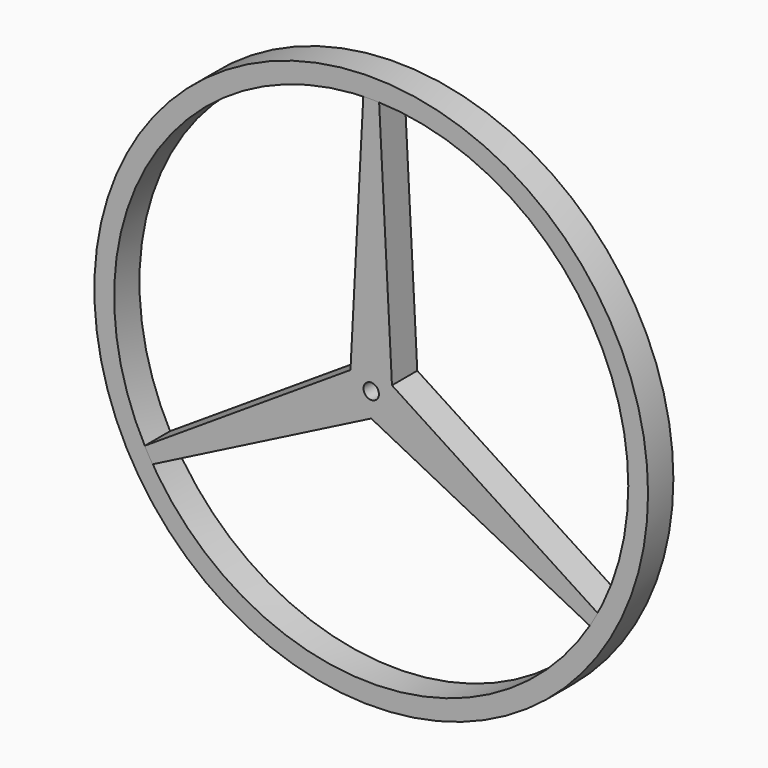
from build123d import *

# Parameters (mm, degrees)
F0_R     = 35
F0_R_2   = 32.5
F1_DEPTH = 4
F0_R_3   = 2.975
F0_R_4   = 0.975
F3_DEPTH = 4


with BuildPart() as f1:
    # F0 (on Front) → F1 (new body)
    with BuildSketch(Plane.XZ):
        Circle(F0_R)
        Circle(F0_R_2, mode=Mode.SUBTRACT)
    extrude(amount=F1_DEPTH)

    # F4 (on Right) → F5 (revolve, cut)
    with BuildSketch(Plane.YZ):
        Polygon((0, 32.5291901827), (2.1413064096, 1.5684039099), (5.6291026995, 1.5684039099), (5.6291026995, 33.8882990181), (0, 33.8882990181), align=None)
    revolve(axis=Axis((0, 0.7535219193, 0), (0, 1, 0)), mode=Mode.SUBTRACT)


with BuildPart() as f1b:
    # F0 (on Front) → F1, piece 2 (new body)
    with BuildSketch(Plane.XZ):
        Circle(F0_R_3)
        Circle(F0_R_4, mode=Mode.SUBTRACT)
    extrude(amount=F1_DEPTH)

    # F2 (on face) → F3 (join)
    with BuildSketch(Plane.XZ.offset(4)):
        with BuildLine():
            Line((2.6230781922, 1.5144349004), (1, 32.4846117416))
            ThreePointArc((1, 32.4846117416), (0, 32.5), (-1, 32.4846117416))
            Line((-1, 32.4846117416), (-2.6230781922, 1.5144349004))
            Line((-2.6230781922, 1.5144349004), (-2.5198255703, 1.5814879371))
            ThreePointArc((-2.5198255703, 1.5814879371), (0, 2.975), (2.5198255703, 1.5814879371))
            Line((2.5198255703, 1.5814879371), (2.6230781922, 1.5144349004))
        make_face()
        with BuildLine():
            Line((28.6324990003, -15.376280467), (2.6230781922, 1.5144349004))
            Line((2.6230781922, 1.5144349004), (2.6295215145, 1.3914889884))
            ThreePointArc((2.6295215145, 1.3914889884), (2.8873388704, 0.7168676637), (2.975, 0))
            ThreePointArc((2.975, 0), (2.1420749793, -2.0644950431), (0.1096959442, -2.9729769255))
            Line((0.1096959442, -2.9729769255), (0, -3.0288698008))
            Line((0, -3.0288698008), (27.6324990003, -17.1083312746))
            ThreePointArc((27.6324990003, -17.1083312746), (28.145825623, -16.25), (28.6324990003, -15.376280467))
        make_face()
        with BuildLine():
            Line((2.6295215145, 1.3914889884), (2.6230781922, 1.5144349004))
            Line((2.6230781922, 1.5144349004), (2.5198255703, 1.5814879371))
            ThreePointArc((2.5198255703, 1.5814879371), (2.5764255763, 1.4875), (2.6295215145, 1.3914889884))
        make_face()
        with BuildLine():
            Line((-2.5198255703, 1.5814879371), (-2.6230781922, 1.5144349004))
            Line((-2.6230781922, 1.5144349004), (-2.6295215145, 1.3914889884))
            ThreePointArc((-2.6295215145, 1.3914889884), (-2.5764255763, 1.4875), (-2.5198255703, 1.5814879371))
        make_face()
        with BuildLine():
            Line((-2.6295215145, 1.3914889884), (-2.6230781922, 1.5144349004))
            Line((-2.6230781922, 1.5144349004), (-28.6324990003, -15.376280467))
            ThreePointArc((-28.6324990003, -15.376280467), (-28.145825623, -16.25), (-27.6324990003, -17.1083312746))
            Line((-27.6324990003, -17.1083312746), (0, -3.0288698008))
            Line((0, -3.0288698008), (-0.1096959442, -2.9729769255))
            ThreePointArc((-0.1096959442, -2.9729769255), (-2.5764255763, -1.4875), (-2.6295215145, 1.3914889884))
        make_face()
        with BuildLine():
            Line((0, -3.0288698008), (0.1096959442, -2.9729769255))
            ThreePointArc((0.1096959442, -2.9729769255), (0, -2.975), (-0.1096959442, -2.9729769255))
            Line((-0.1096959442, -2.9729769255), (0, -3.0288698008))
        make_face()
    extrude(amount=-F3_DEPTH)


solid = Compound([f1.part, f1b.part])
